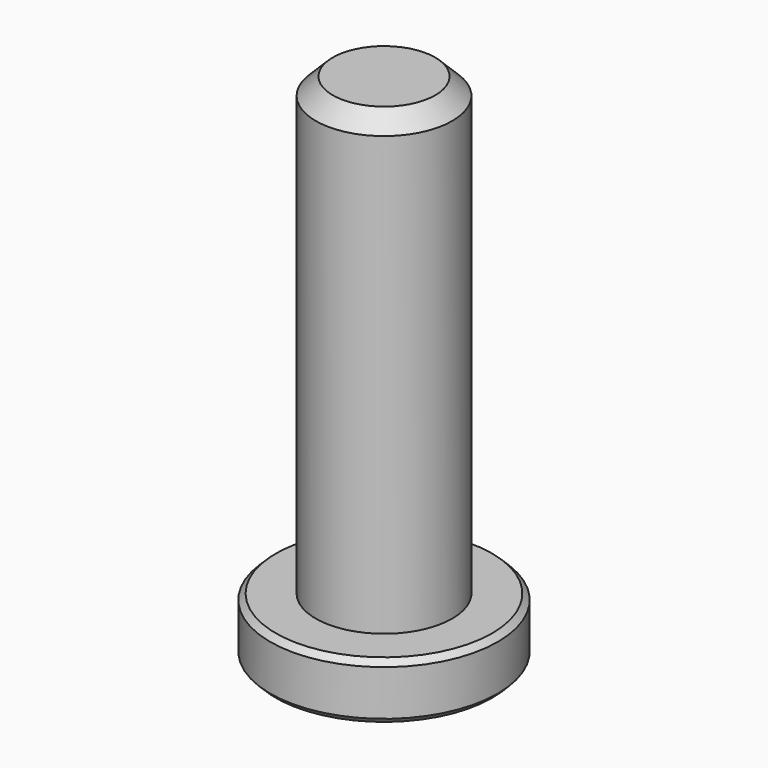
from build123d import *

# Parameters (mm, degrees)
F1_R     = 6
F2_DEPTH = 40
F0_R     = 10
F3_DEPTH = 5
F4_SIZE  = 0.5
F5_SIZE  = 1.5


# Not quite as in the source:
# - the program builds the solid bodies; features that only make, move or delete a surface that nothing else refers to are left out


with BuildPart() as f2:
    # F1 (on face) → F2 (new body)
    with BuildSketch(Plane.XY):
        Circle(F1_R)
    extrude(amount=F2_DEPTH)

    # F0 (on Top) → F3 (join)
    with BuildSketch(Plane.XY):
        Circle(F0_R)
    extrude(amount=-F3_DEPTH)

    # F4
    f4_edges = [f2.edges().sort_by_distance(p)[0] for p in [
        (-10, 0, 0),
        (-10, 0, -5),
    ]]
    chamfer(f4_edges, length=F4_SIZE)

    # F5
    f5_edges = [f2.edges().sort_by_distance(p)[0] for p in [
        (-6, 0, 40),
    ]]
    chamfer(f5_edges, length=F5_SIZE)


solid = f2.part
